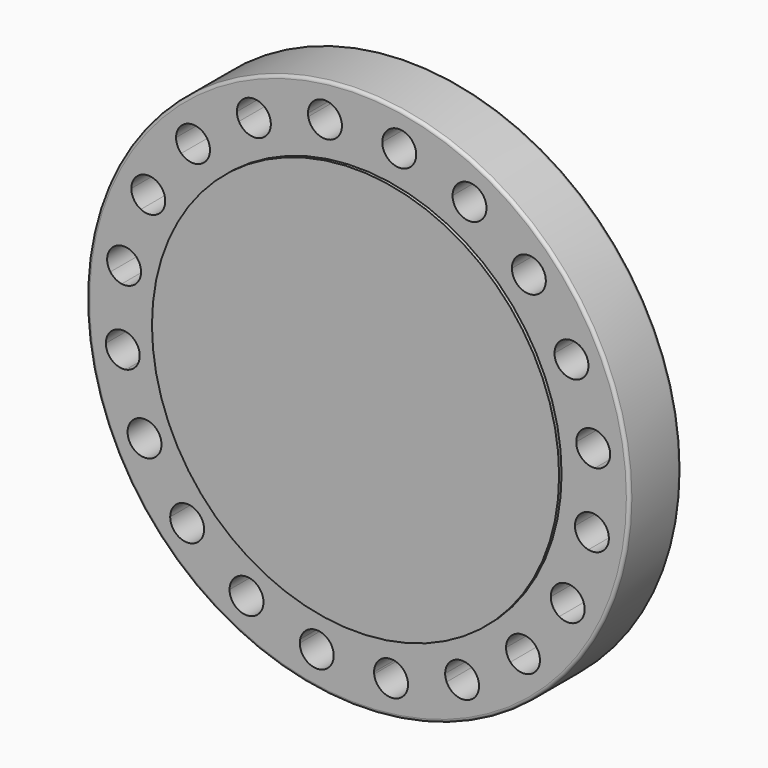
from build123d import *

# Parameters (mm, degrees)
F0_R            = 279.4
F1_DEPTH        = 66.548
F2_R            = 3.175
F3_R            = 209.55
F4_DEPTH        = 3.175
F6_DEPTH        = 76.2
F6_COPIES_COUNT = 8
F6_COPIES_ANGLE = 252


# Not quite as in the source:
# - a pattern or mirror of a feature is missing from the dataset's text; its kind, count and spacing are read off the source's solid


with BuildPart() as f1:
    # F0 (on Front) → F1 (new body)
    with BuildSketch(Plane.XZ):
        Circle(F0_R)
    extrude(amount=F1_DEPTH)

    # F2
    f2_edges = [f1.edges().sort_by_distance(p)[0] for p in [
        (-279.4, -66.548, 0),
        (-279.4, 0, 0),
    ]]
    fillet(f2_edges, radius=F2_R)

    # F3 (on face) → F4 (join)
    with BuildSketch(Plane.XZ.offset(66.548)):
        Circle(F3_R)
    extrude(amount=F4_DEPTH)

    # F5 (on face) → F6 (cut)
    with BuildSketch(Plane(origin=(0, 0, 0), x_dir=(-1, 0, 0), z_dir=(0, 1, 0))):
        with BuildLine():
            ThreePointArc((259.5582861056, -34.0243438572), (255.0681882926, -22.3343614899), (243.9069546527, -16.6560228461))
            ThreePointArc((243.9069546527, -16.6560228461), (242.0957861056, -34.0243438572), (239.0494349763, -51.2190712772))
            ThreePointArc((239.0494349763, -51.2190712772), (253.31501067, -47.405969559), (259.5582861056, -34.0243438572))
        make_face()
        with BuildLine():
            ThreePointArc((239.0494349763, -51.2190712772), (242.0957861056, -34.0243438572), (243.9069546527, -16.6560228461))
            ThreePointArc((243.9069546527, -16.6560228461), (224.8032299552, -31.5940335817), (239.0494349763, -51.2190712772))
        make_face()
        with BuildLine():
            ThreePointArc((207.1150359511, 129.8899053352), (200.4401404239, 106.5759131469), (223.5008701244, 99.0726333486))
            ThreePointArc((223.5008701244, 99.0726333486), (215.8586127642, 114.7740603121), (207.1150359511, 129.8899053352))
        make_face()
        with BuildLine():
            ThreePointArc((207.1150359511, 129.8899053352), (215.8586127642, 114.7740603121), (223.5008701244, 99.0726333486))
            ThreePointArc((223.5008701244, 99.0726333486), (230.6638791482, 105.5143090439), (233.3211127642, 114.7740603121))
            ThreePointArc((233.3211127642, 114.7740603121), (224.5836971807, 129.9005869515), (207.1150359511, 129.8899053352))
        make_face()
        with BuildLine():
            ThreePointArc((237.195174469, -107.1707861113), (234.3740809966, -97.6540576217), (226.822304474, -91.2122130973))
            ThreePointArc((226.822304474, -91.2122130973), (219.732674469, -107.1707861113), (211.5219593902, -122.5825694002))
            ThreePointArc((211.5219593902, -122.5825694002), (228.7204243038, -122.142735188), (237.195174469, -107.1707861113))
        make_face()
        with BuildLine():
            ThreePointArc((211.5219593902, -122.5825694002), (219.732674469, -107.1707861113), (226.822304474, -91.2122130973))
            ThreePointArc((226.822304474, -91.2122130973), (204.0374834355, -99.5157299605), (211.5219593902, -122.5825694002))
        make_face()
        with BuildLine():
            ThreePointArc((156.8399164176, 187.5347067695), (157.6961333238, 163.2991264244), (181.9468315473, 163.2892406587))
            ThreePointArc((181.9468315473, 163.2892406587), (169.826605118, 175.8605976878), (156.8399164176, 187.5347067695))
        make_face()
        with BuildLine():
            ThreePointArc((156.8399164176, 187.5347067695), (169.826605118, 175.8605976878), (181.9468315473, 163.2892406587))
            ThreePointArc((181.9468315473, 163.2892406587), (185.8981383409, 169.03090325), (187.289105118, 175.8605976878))
            ThreePointArc((187.289105118, 175.8605976878), (176.0779591641, 192.1657955964), (156.8399164176, 187.5347067695))
        make_face()
        with BuildLine():
            ThreePointArc((193.3230976878, -169.826605118), (191.8104885352, -162.7174639458), (187.5347067695, -156.8399164176))
            ThreePointArc((187.5347067695, -156.8399164176), (175.8605976878, -169.826605118), (163.2892406587, -181.9468315473))
            ThreePointArc((163.2892406587, -181.9468315473), (182.3955645634, -186.0202184944), (193.3230976878, -169.826605118))
        make_face()
        with BuildLine():
            ThreePointArc((163.2892406587, -181.9468315473), (175.8605976878, -169.826605118), (187.5347067695, -156.8399164176))
            ThreePointArc((187.5347067695, -156.8399164176), (163.2991264244, -157.6961333238), (163.2892406587, -181.9468315473))
        make_face()
        with BuildLine():
            ThreePointArc((91.2122130973, 226.822304474), (99.5157299605, 204.0374834355), (122.5825694002, 211.5219593902))
            ThreePointArc((122.5825694002, 211.5219593902), (107.1707861113, 219.732674469), (91.2122130973, 226.822304474))
        make_face()
        with BuildLine():
            ThreePointArc((91.2122130973, 226.822304474), (107.1707861113, 219.732674469), (122.5825694002, 211.5219593902))
            ThreePointArc((122.5825694002, 211.5219593902), (124.1128516868, 215.501206605), (124.6332861113, 219.732674469))
            ThreePointArc((124.6332861113, 219.732674469), (110.7944807034, 236.8150555604), (91.2122130973, 226.822304474))
        make_face()
        with BuildLine():
            ThreePointArc((132.2365603121, -215.8586127642), (131.639696232, -211.332109559), (129.8899053352, -207.1150359511))
            ThreePointArc((129.8899053352, -207.1150359511), (114.7740603121, -215.8586127642), (99.0726333486, -223.5008701244))
            ThreePointArc((99.0726333486, -223.5008701244), (118.6953316557, -232.8751499354), (132.2365603121, -215.8586127642))
        make_face()
        with BuildLine():
            ThreePointArc((99.0726333486, -223.5008701244), (114.7740603121, -215.8586127642), (129.8899053352, -207.1150359511))
            ThreePointArc((129.8899053352, -207.1150359511), (106.5759131469, -200.4401404239), (99.0726333486, -223.5008701244))
        make_face()
        with BuildLine():
            ThreePointArc((31.5940335817, 224.8032299552), (44.2827839326, 227.9641438277), (51.2190712772, 239.0494349763))
            ThreePointArc((51.2190712772, 239.0494349763), (42.6489158097, 240.7261838796), (34.0243438572, 242.0957861056))
            Line((34.0243438572, 242.0957861056), (31.5940335817, 224.8032299552))
        make_face()
        with BuildLine():
            ThreePointArc((34.0243438572, 242.0957861056), (42.6489158097, 240.7261838796), (51.2190712772, 239.0494349763))
            ThreePointArc((51.2190712772, 239.0494349763), (51.4197719034, 240.5667375977), (51.4868438572, 242.0957861056))
            ThreePointArc((51.4868438572, 242.0957861056), (47.2034599019, 253.5522168993), (36.4546541327, 259.388342256))
            Line((36.4546541327, 259.388342256), (34.0243438572, 242.0957861056))
        make_face()
        with BuildLine():
            ThreePointArc((59.9151382351, -240.7608754177), (59.8187312974, -238.9284677109), (59.5305749705, -237.1162927103))
            ThreePointArc((59.5305749705, -237.1162927103), (42.4526382351, -240.7608754177), (25.1581064067, -243.1770863117))
            ThreePointArc((25.1581064067, -243.1770863117), (43.6636593323, -258.1813327639), (59.9151382351, -240.7608754177))
        make_face()
        with BuildLine():
            ThreePointArc((25.1581064067, -243.1770863117), (42.4526382351, -240.7608754177), (59.5305749705, -237.1162927103))
            ThreePointArc((59.5305749705, -237.1162927103), (39.4203069326, -223.5636700307), (25.1581064067, -243.1770863117))
        make_face()
        with BuildLine():
            Line((31.5940335817, 224.8032299552), (34.0243438572, 242.0957861056))
            ThreePointArc((34.0243438572, 242.0957861056), (25.3563596593, 243.1564941552), (16.6560228461, 243.9069546527))
            ThreePointArc((16.6560228461, 243.9069546527), (20.2680898419, 231.3391889803), (31.5940335817, 224.8032299552))
        make_face()
        with BuildLine():
            ThreePointArc((16.6560228461, 243.9069546527), (25.3563596593, 243.1564941552), (34.0243438572, 242.0957861056))
            Line((34.0243438572, 242.0957861056), (36.4546541327, 259.388342256))
            ThreePointArc((36.4546541327, 259.388342256), (23.267746732, 255.852040121), (16.6560228461, 243.9069546527))
        make_face()
        with BuildLine():
            ThreePointArc((-51.2190712772, -239.0494349763), (-36.4546541327, -259.388342256), (-16.6560228461, -243.9069546527))
            ThreePointArc((-16.6560228461, -243.9069546527), (-34.0243438572, -242.0957861056), (-51.2190712772, -239.0494349763))
        make_face()
        with BuildLine():
            ThreePointArc((-51.2190712772, -239.0494349763), (-34.0243438572, -242.0957861056), (-16.6560228461, -243.9069546527))
            ThreePointArc((-16.6560228461, -243.9069546527), (-16.5854044986, -243.0025938564), (-16.5618438572, -242.0957861056))
            ThreePointArc((-16.5618438572, -242.0957861056), (-32.4952953494, -224.7003580594), (-51.2190712772, -239.0494349763))
        make_face()
        with BuildLine():
            ThreePointArc((-24.9901382351, 240.7608754177), (-25.0321808889, 241.9718965148), (-25.1581064067, 243.1770863117))
            ThreePointArc((-25.1581064067, 243.1770863117), (-42.4526382351, 240.7608754177), (-59.5305749705, 237.1162927103))
            ThreePointArc((-59.5305749705, 237.1162927103), (-40.6202305284, 223.3947823554), (-24.9901382351, 240.7608754177))
        make_face()
        with BuildLine():
            ThreePointArc((-59.5305749705, 237.1162927103), (-42.4526382351, 240.7608754177), (-25.1581064067, 243.1770863117))
            ThreePointArc((-25.1581064067, 243.1770863117), (-45.4849695376, 257.9580808046), (-59.5305749705, 237.1162927103))
        make_face()
        with BuildLine():
            ThreePointArc((-122.5825694002, -211.5219593902), (-114.8258422621, -235.4278655025), (-91.2122130973, -226.822304474))
            ThreePointArc((-91.2122130973, -226.822304474), (-107.1707861113, -219.732674469), (-122.5825694002, -211.5219593902))
        make_face()
        with BuildLine():
            ThreePointArc((-122.5825694002, -211.5219593902), (-107.1707861113, -219.732674469), (-91.2122130973, -226.822304474))
            ThreePointArc((-91.2122130973, -226.822304474), (-90.0884050198, -223.3563690611), (-89.7082861113, -219.732674469))
            ThreePointArc((-89.7082861113, -219.732674469), (-102.9393182473, -202.7906088934), (-122.5825694002, -211.5219593902))
        make_face()
        with BuildLine():
            ThreePointArc((-97.3115603121, 215.8586127642), (-97.7575231408, 219.7798841078), (-99.0726333486, 223.5008701244))
            ThreePointArc((-99.0726333486, 223.5008701244), (-114.7740603121, 215.8586127642), (-129.8899053352, 207.1150359511))
            ThreePointArc((-129.8899053352, 207.1150359511), (-110.2475571069, 198.9929768443), (-97.3115603121, 215.8586127642))
        make_face()
        with BuildLine():
            ThreePointArc((-129.8899053352, 207.1150359511), (-114.7740603121, 215.8586127642), (-99.0726333486, 223.5008701244))
            ThreePointArc((-99.0726333486, 223.5008701244), (-122.9722074772, 231.2770851045), (-129.8899053352, 207.1150359511))
        make_face()
        with BuildLine():
            ThreePointArc((-181.9468315473, -163.2892406587), (-181.9570769121, -188.4220689512), (-156.8399164176, -187.5347067695))
            ThreePointArc((-156.8399164176, -187.5347067695), (-169.826605118, -175.8605976878), (-181.9468315473, -163.2892406587))
        make_face()
        with BuildLine():
            ThreePointArc((-181.9468315473, -163.2892406587), (-169.826605118, -175.8605976878), (-156.8399164176, -187.5347067695))
            ThreePointArc((-156.8399164176, -187.5347067695), (-153.5214072093, -182.1119517339), (-152.364105118, -175.8605976878))
            ThreePointArc((-152.364105118, -175.8605976878), (-162.9969106801, -159.7890644649), (-181.9468315473, -163.2892406587))
        make_face()
        with BuildLine():
            ThreePointArc((-158.3980976878, 169.826605118), (-159.6669843114, 176.3615719936), (-163.2892406587, 181.9468315473))
            ThreePointArc((-163.2892406587, 181.9468315473), (-175.8605976878, 169.826605118), (-187.5347067695, 156.8399164176))
            ThreePointArc((-187.5347067695, 156.8399164176), (-168.7514565156, 153.8767142706), (-158.3980976878, 169.826605118))
        make_face()
        with BuildLine():
            ThreePointArc((-187.5347067695, 156.8399164176), (-175.8605976878, 169.826605118), (-163.2892406587, 181.9468315473))
            ThreePointArc((-163.2892406587, 181.9468315473), (-188.4220689512, 181.9570769121), (-187.5347067695, 156.8399164176))
        make_face()
        with BuildLine():
            ThreePointArc((-223.5008701244, -99.0726333486), (-231.2770851045, -122.9722074772), (-207.1150359511, -129.8899053352))
            ThreePointArc((-207.1150359511, -129.8899053352), (-215.8586127642, -114.7740603121), (-223.5008701244, -99.0726333486))
        make_face()
        with BuildLine():
            ThreePointArc((-223.5008701244, -99.0726333486), (-215.8586127642, -114.7740603121), (-207.1150359511, -129.8899053352))
            ThreePointArc((-207.1150359511, -129.8899053352), (-200.7320861247, -123.4991447286), (-198.3961127642, -114.7740603121))
            ThreePointArc((-198.3961127642, -114.7740603121), (-206.598861496, -99.9687939281), (-223.5008701244, -99.0726333486))
        make_face()
        with BuildLine():
            ThreePointArc((-202.270174469, 107.1707861113), (-204.7607253922, 116.1585359461), (-211.5219593902, 122.5825694002))
            ThreePointArc((-211.5219593902, 122.5825694002), (-219.732674469, 107.1707861113), (-226.822304474, 91.2122130973))
            ThreePointArc((-226.822304474, 91.2122130973), (-210.2159459794, 92.5293795837), (-202.270174469, 107.1707861113))
        make_face()
        with BuildLine():
            ThreePointArc((-226.822304474, 91.2122130973), (-219.732674469, 107.1707861113), (-211.5219593902, 122.5825694002))
            ThreePointArc((-211.5219593902, 122.5825694002), (-235.4278655025, 114.8258422621), (-226.822304474, 91.2122130973))
        make_face()
        with BuildLine():
            ThreePointArc((-243.1770863117, -25.1581064067), (-257.9580808046, -45.4849695376), (-237.1162927103, -59.5305749705))
            ThreePointArc((-237.1162927103, -59.5305749705), (-240.7608754177, -42.4526382351), (-243.1770863117, -25.1581064067))
        make_face()
        with BuildLine():
            ThreePointArc((-243.1770863117, -25.1581064067), (-240.7608754177, -42.4526382351), (-237.1162927103, -59.5305749705))
            ThreePointArc((-237.1162927103, -59.5305749705), (-227.1854853353, -53.4366124868), (-223.2983754177, -42.4526382351))
            ThreePointArc((-223.2983754177, -42.4526382351), (-229.2990731267, -29.2781934843), (-243.1770863117, -25.1581064067))
        make_face()
        with BuildLine():
            ThreePointArc((-224.6332861056, 34.0243438572), (-228.7141604038, 45.2435684217), (-239.0494349763, 51.2190712772))
            ThreePointArc((-239.0494349763, 51.2190712772), (-242.0957861056, 34.0243438572), (-243.9069546527, 16.6560228461))
            ThreePointArc((-243.9069546527, 16.6560228461), (-230.4058037383, 21.0519416702), (-224.6332861056, 34.0243438572))
        make_face()
        with BuildLine():
            ThreePointArc((-243.9069546527, 16.6560228461), (-242.0957861056, 34.0243438572), (-239.0494349763, 51.2190712772))
            ThreePointArc((-239.0494349763, 51.2190712772), (-259.388342256, 36.4546541327), (-243.9069546527, 16.6560228461))
        make_face()
    f6 = extrude(amount=-F6_DEPTH, mode=Mode.SUBTRACT)

    # F6_copies: F6 ×8 about axis
    f6_copies_axis = Axis((0, 0, 0), (0, -1, 0))
    for i in range(1, F6_COPIES_COUNT):
        add(f6.rotate(f6_copies_axis, i * F6_COPIES_ANGLE / (F6_COPIES_COUNT - 1)), mode=Mode.SUBTRACT)


solid = f1.part
